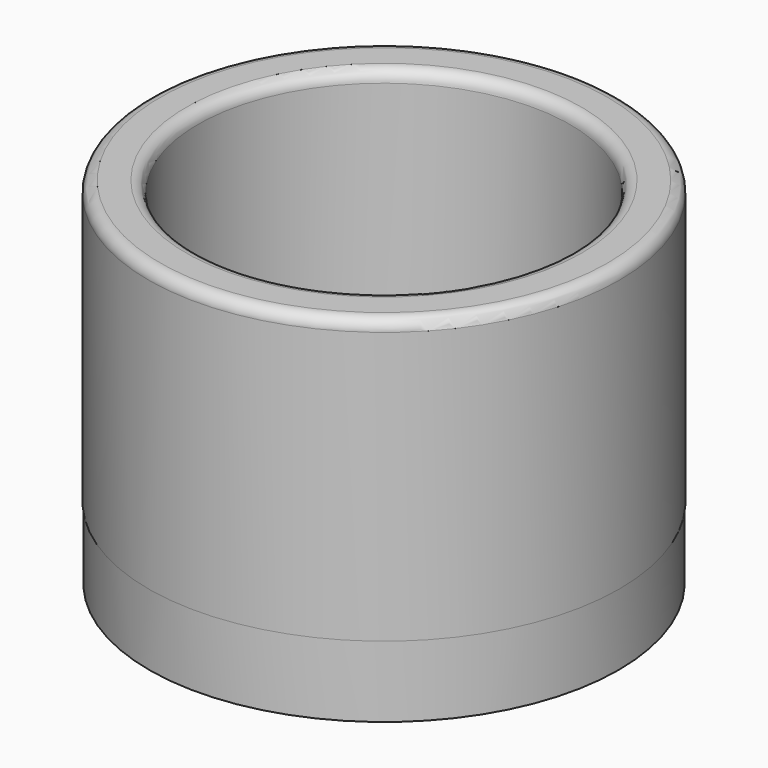
from build123d import *

# Parameters (mm, degrees)
F0_R     = 50.2290121712
F0_R_2   = 39.7205191913
F1_DEPTH = 60.452
F2_R     = 50.1012725797
F3_DEPTH = 15.24
F4_R     = 2.4528409794


# Not quite as in the source:
# - a feature names something its author has since deleted; it is built from what else it names


with BuildPart() as f1:
    # F0 (on Top) → F1 (new body)
    with BuildSketch(Plane.XY):
        Circle(F0_R)
        Circle(F0_R_2, mode=Mode.SUBTRACT)
    extrude(amount=F1_DEPTH)

    # F2 (on face) → F3 (join)
    with BuildSketch(Plane(origin=(0, 0, 0), x_dir=(1, 0, 0), z_dir=(0, 0, -1))):
        Circle(F2_R)
    extrude(amount=F3_DEPTH)

    # F4
    f4_edges = [f1.edges().sort_by_distance(p)[0] for p in [
        (-50.229012, 0, 60.452),
        (-39.720519, 0, 60.452),
    ]]
    fillet(f4_edges, radius=F4_R)


solid = f1.part
